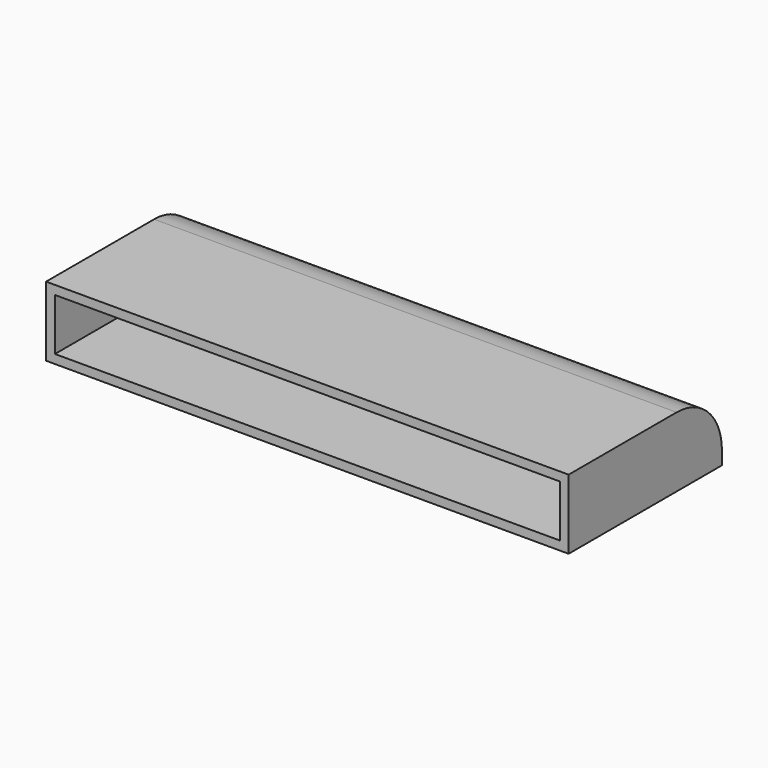
from build123d import *

# Parameters (mm, degrees)
F0_W     = 150
F0_H     = 50
F1_DEPTH = 20
F2_T     = -2.54
F3_DEPTH = 5
F4_R     = 16.256


with BuildPart() as f1:
    # F0 (on Top) → F1 (new body)
    with BuildSketch(Plane.XY):
        with Locations((1.6509965062, -8.4789711357)):
            Rectangle(F0_W, F0_H)
    extrude(amount=F1_DEPTH)

    # F2
    f2_openings = [f1.faces().sort_by_distance(p)[0] for p in [
        (1.650997, -33.478971, 10),
    ]]
    offset(amount=F2_T, openings=f2_openings)

    # F3 (add): a face of the model
    f3_faces = [f1.faces().sort_by_distance(p)[0] for p in [
        (1.6509965062, 16.5210288643, 10),
    ]]
    extrude(f3_faces, amount=F3_DEPTH)

    # F4
    f4_edges = [f1.edges().sort_by_distance(p)[0] for p in [
        (1.650997, 21.521029, 20),
    ]]
    fillet(f4_edges, radius=F4_R)


solid = f1.part
